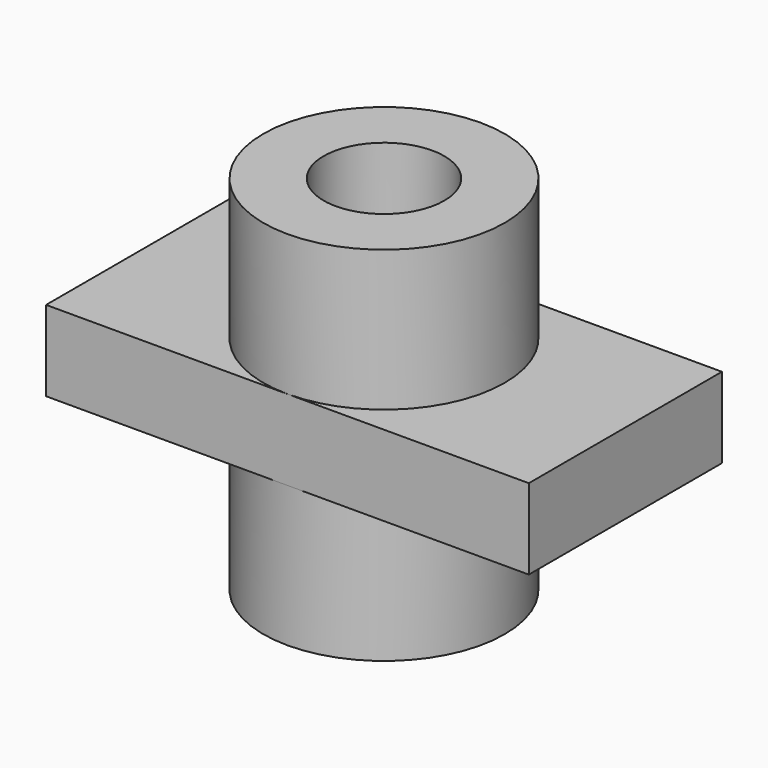
from build123d import *
from build123d import SkipClean  # not in build123d's __all__

# Parameters (mm, degrees)
F1_DEPTH      = 28.575
F2_W          = 76.2
F2_H          = 12.7
F3_DEPTH      = 19.05
F3_DEPTH_BACK = 19.05
F4_R          = 9.525
F5_DEPTH      = 34.926


with BuildPart() as f1:
    # F0 (on Top) → F1 (new body, symmetric)
    with BuildSketch(Plane.XY):
        with BuildLine():
            ThreePointArc((0, 19.05), (-19.05, 0), (0, -19.05))
            Line((0, -19.05), (0, -9.525))
            ThreePointArc((0, -9.525), (-9.525, 0), (0, 9.525))
            Line((0, 9.525), (0, 19.05))
        make_face()
        with BuildLine():
            Line((0, -9.525), (0, -19.05))
            ThreePointArc((0, -19.05), (13.4703841816, -13.4703841816), (19.05, 0))
            ThreePointArc((19.05, 0), (13.4703841816, 13.4703841816), (0, 19.05))
            Line((0, 19.05), (0, 9.525))
            ThreePointArc((0, 9.525), (6.7351920908, 6.7351920908), (9.525, 0))
            ThreePointArc((9.525, 0), (6.7351920908, -6.7351920908), (0, -9.525))
        make_face()
    extrude(amount=F1_DEPTH, both=True)

    # F2 (on Front) → F3 (join, two sides)
    with BuildSketch(Plane.XZ) as f3_sk:
        Rectangle(F2_W, F2_H)
    extrude(amount=-F3_DEPTH)
    extrude(f3_sk.sketch, amount=F3_DEPTH_BACK)

    # F4 (on face) → F5 (cut, through all)
    with BuildSketch(Plane.XY.offset(6.35)):
        Circle(F4_R)
    with SkipClean():  # cleaning this boolean's faces spoils the solid; the shape is the same uncleaned
        extrude(amount=-F5_DEPTH, mode=Mode.SUBTRACT)


solid = f1.part
